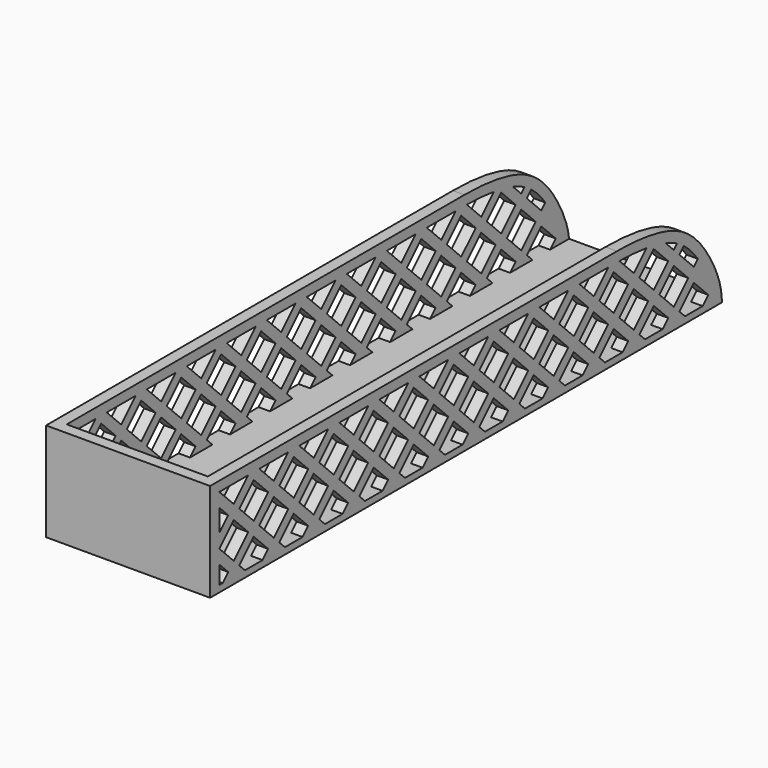
from build123d import *

# Parameters (mm, degrees)
F0_W     = 50
F0_H     = 195
F1_DEPTH = 2
F3_DEPTH = 28
F5_DEPTH = 50.001
F7_DEPTH = 50.0010001
F9_D     = 3.2


# Not quite as in the source:
# - ends of sketch curves that miss each other by under 0.0002 mm in the source are joined
# - the dataset's text gives a spline's control points without its knots; the knots are read off the source's solid


with BuildPart() as f1:
    # F0 (on Top) → F1 (new body)
    with BuildSketch(Plane.XY):
        with Locations((25, 97.5)):
            Rectangle(F0_W, F0_H)
    extrude(amount=F1_DEPTH)

    # F2 (on face) → F3 (join)
    with BuildSketch(Plane.XY.offset(2)):
        Polygon((50, 0), (50, 195), (46.5, 195), (46.5, 3.5), (3.5, 3.5), (3.5, 195), (0, 195), (0, 0), align=None)
    extrude(amount=F3_DEPTH)

    # F4 (on face) → F5 (cut, through all)
    with BuildSketch(Plane.YZ.offset(50)):
        with BuildLine():
            add(Edge.make_bspline(
                [(195, 0), (195, 4.6234254886), (190.8875835755, 14.6924515974), (179.2887315108, 28.7129007105), (161.6677078594, 30), (155, 30)],
                knots=[0, 0, 0, 0, 0.2989346859, 0.625276018, 1, 1, 1, 1], degree=3))
            Line((195, 0), (195, 30))
            Line((195, 30), (155, 30))
        make_face()
    extrude(amount=-F5_DEPTH, mode=Mode.SUBTRACT)

    # F6 (on face) → F7 (cut, through all)
    with BuildSketch(Plane.YZ.offset(50)):
        Polygon((14.5, 27), (3.5, 27), (9, 21.5), align=None)
        Polygon((6.8786796564, 19.3786796564), (3.5, 22.7573593129), (3.5, 16), align=None)
        Polygon((9, 17.2573593129), (3.5, 11.7573593129), (9, 6.2573593129), (14.5, 11.7573593129), align=None)
        Polygon((6.8786796564, 4.1360389693), (3.5, 7.5147186258), (3.5, 2), (4.7426406871, 2), align=None)
        Polygon((11.1213203436, 4.1360389693), (13.2573593129, 2), (19.9852813742, 2), (22.1213203436, 4.1360389693), (16.6213203436, 9.6360389693), align=None)
        Polygon((16.6213203436, 24.8786796564), (11.1213203436, 19.3786796564), (16.6213203436, 13.8786796564), (22.1213203436, 19.3786796564), align=None)
        Polygon((29.743, 27), (18.743, 27), (24.243, 21.5), align=None)
        Polygon((24.243, 6.2573593129), (29.743, 11.7573593129), (24.243, 17.2573593129), (18.743, 11.7573593129), align=None)
        Polygon((31.8643203436, 24.8786796564), (26.3643203436, 19.3786796564), (31.8643203436, 13.8786796564), (37.3643203436, 19.3786796564), align=None)
        Polygon((26.3643203436, 4.1360389693), (28.5003593129, 2), (35.2282813742, 2), (37.3643203436, 4.1360389693), (31.8643203436, 9.6360389693), align=None)
        Polygon((39.486, 6.2573593129), (44.986, 11.7573593129), (39.486, 17.2573593129), (33.986, 11.7573593129), align=None)
        Polygon((44.986, 27), (33.986, 27), (39.486, 21.5), align=None)
        Polygon((47.1073203436, 24.8786796564), (41.6073203436, 19.3786796564), (47.1073203436, 13.8786796564), (52.6073203436, 19.3786796564), align=None)
        Polygon((41.6073203436, 4.1360389693), (43.7433593129, 2), (50.4712813742, 2), (52.6073203436, 4.1360389693), (47.1073203436, 9.6360389693), align=None)
        Polygon((54.729, 6.2573593129), (60.229, 11.7573593129), (54.729, 17.2573593129), (49.229, 11.7573593129), align=None)
        Polygon((60.229, 27), (49.229, 27), (54.729, 21.5), align=None)
        Polygon((62.3503203436, 24.8786796564), (56.8503203436, 19.3786796564), (62.3503203436, 13.8786796564), (67.8503203436, 19.3786796564), align=None)
        Polygon((56.8503203436, 4.1360389693), (58.9863593129, 2), (65.7142813742, 2), (67.8503203436, 4.1360389693), (62.3503203436, 9.6360389693), align=None)
        Polygon((69.972, 6.2573593129), (75.472, 11.7573593129), (69.972, 17.2573593129), (64.472, 11.7573593129), align=None)
        Polygon((75.472, 27), (64.472, 27), (69.972, 21.5), align=None)
        Polygon((77.5933203436, 24.8786796564), (72.0933203436, 19.3786796564), (77.5933203436, 13.8786796564), (83.0933203436, 19.3786796564), align=None)
        Polygon((74.2293593129, 2), (80.9572813742, 2), (83.0933203436, 4.1360389693), (77.5933203436, 9.6360389693), (72.0933203436, 4.1360389693), align=None)
        Polygon((85.215, 6.2573593129), (90.715, 11.7573593129), (85.215, 17.2573593129), (79.715, 11.7573593129), align=None)
        Polygon((90.715, 27), (79.715, 27), (85.215, 21.5), align=None)
        Polygon((92.8363203436, 24.8786796564), (87.3363203436, 19.3786796564), (92.8363203436, 13.8786796564), (98.3363203436, 19.3786796564), align=None)
        Polygon((89.4723593129, 2), (96.2002813742, 2), (98.3363203436, 4.1360389693), (92.8363203436, 9.6360389693), (87.3363203436, 4.1360389693), align=None)
        Polygon((100.458, 6.2573593129), (105.958, 11.7573593129), (100.458, 17.2573593129), (94.958, 11.7573593129), align=None)
        Polygon((105.958, 27), (94.958, 27), (100.458, 21.5), align=None)
        Polygon((108.0793203436, 24.8786796564), (102.5793203436, 19.3786796564), (108.0793203436, 13.8786796564), (113.5793203436, 19.3786796564), align=None)
        Polygon((104.7153593129, 2), (111.4432813742, 2), (113.5793203436, 4.1360389693), (108.0793203436, 9.6360389693), (102.5793203436, 4.1360389693), align=None)
        Polygon((115.701, 6.2573593129), (121.201, 11.7573593129), (115.701, 17.2573593129), (110.201, 11.7573593129), align=None)
        Polygon((115.701, 21.5), (121.201, 27), (110.201, 27), align=None)
        Polygon((123.3223203436, 24.8786796564), (117.8223203436, 19.3786796564), (123.3223203436, 13.8786796564), (128.8223203436, 19.3786796564), align=None)
        Polygon((130.944, 6.2573593129), (136.444, 11.7573593129), (130.944, 17.2573593129), (125.444, 11.7573593129), align=None)
        Polygon((119.9583593129, 2), (126.6862813742, 2), (128.8223203436, 4.1360389693), (123.3223203436, 9.6360389693), (117.8223203436, 4.1360389693), align=None)
        Polygon((130.944, 21.5), (136.444, 27), (125.444, 27), align=None)
        Polygon((138.5653203436, 24.8786796564), (133.0653203436, 19.3786796564), (138.5653203436, 13.8786796564), (144.0653203436, 19.3786796564), align=None)
        Polygon((146.187, 6.2573593129), (151.687, 11.7573593129), (146.187, 17.2573593129), (140.687, 11.7573593129), align=None)
        Polygon((135.2013593129, 2), (141.9292813742, 2), (144.0653203436, 4.1360389693), (138.5653203436, 9.6360389693), (133.0653203436, 4.1360389693), align=None)
        Polygon((150.4443593129, 2), (157.1722813742, 2), (159.3083203436, 4.1360389693), (153.8083203436, 9.6360389693), (148.3083203436, 4.1360389693), align=None)
        Polygon((146.187, 21.5), (151.687, 27), (140.687, 27), align=None)
        Polygon((153.8083203436, 24.8786796564), (148.3083203436, 19.3786796564), (153.8083203436, 13.8786796564), (159.3083203436, 19.3786796564), align=None)
        Polygon((161.43, 6.2573593129), (166.93, 11.7573593129), (161.43, 17.2573593129), (155.93, 11.7573593129), align=None)
        Polygon((165.6873593129, 2), (172.4152813742, 2), (174.5513203436, 4.1360389693), (169.0513203436, 9.6360389693), (163.5513203436, 4.1360389693), align=None)
        Polygon((180.9303593129, 2), (187.6582813742, 2), (189.7943203436, 4.1360389693), (184.2943203436, 9.6360389693), (178.7943203436, 4.1360389693), align=None)
        Polygon((176.673, 6.2573593129), (182.173, 11.7573593129), (176.673, 17.2573593129), (171.173, 11.7573593129), align=None)
        Polygon((169.0513203436, 24.8786796564), (163.5513203436, 19.3786796564), (169.0513203436, 13.8786796564), (174.5513203436, 19.3786796564), align=None)
        with BuildLine():
            Line((161.43, 21.5), (166.1919188793, 26.2619188793))
            add(Edge.make_bspline(
                [(166.1919188793, 26.2619188793), (166.119628747, 26.2723011534), (164.7673946206, 26.4640860842), (161.1979644468, 26.8486616211), (157.8526668959, 26.9760954229), (155.9346811245, 26.9953188755)],
                knots=[0.8089686708, 0.8089686708, 0.8089686708, 0.8089686708, 0.8125, 0.875, 0.9822650856, 0.9822650856, 0.9822650856, 0.9822650856], degree=3))
            Line((155.9346811245, 26.9953188755), (161.43, 21.5))
        make_face()
        with BuildLine():
            Line((176.673, 21.5), (177.9224878354, 22.7494878354))
            add(Edge.make_bspline(
                [(177.9224878354, 22.7494878354), (177.4771181354, 22.9988507452), (176.5450084907, 23.4777533512), (175.0832558256, 24.0960693971), (174.0474190582, 24.4616023471), (173.5497894669, 24.623201445)],
                knots=[0.5945932873, 0.5945932873, 0.5945932873, 0.5945932873, 0.625, 0.65625, 0.683753381, 0.683753381, 0.683753381, 0.683753381], degree=3))
            Line((173.5497894669, 24.623201445), (176.673, 21.5))
        make_face()
        with BuildLine():
            Line((184.2943203436, 13.8786796564), (185.8272365841, 15.411595897))
            add(Edge.make_bspline(
                [(185.8272365841, 15.411595897), (185.7907825855, 15.4624594773), (185.1581159252, 16.340691239), (183.8590605827, 17.9751180761), (182.0779172773, 19.7694121048), (180.897672102, 20.7441925664), (180.4800012881, 21.0643768001)],
                knots=[0.3711666916, 0.3711666916, 0.3711666916, 0.3711666916, 0.375, 0.4375, 0.5, 0.5324946243, 0.5324946243, 0.5324946243, 0.5324946243], degree=3))
            Line((180.4800012881, 21.0643768001), (178.7943203436, 19.3786796564))
            Line((178.7943203436, 19.3786796564), (184.2943203436, 13.8786796564))
        make_face()
    extrude(amount=-F7_DEPTH, mode=Mode.SUBTRACT)

    # F9 (through all)
    with Locations(Plane.XY.offset(2)):
        with Locations((9.75, 42), (40.25, 42), (9.75, 11.5), (40.25, 11.5)):
            Hole(F9_D / 2)


solid = f1.part
